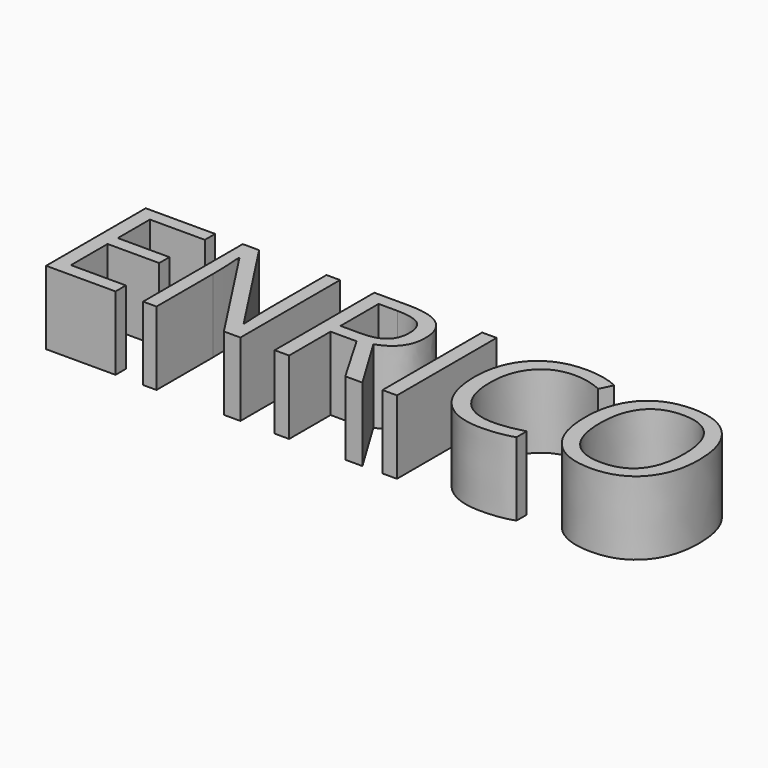
from build123d import *

# Parameters (mm, degrees)
F0_TEXT_SIZE = 60.3270251304
F1_DEPTH     = 25.4


# Not quite as in the source:
# - Text() gives the source's letters only with a copy of the font that has no kerning and outlines rounded to 1/6400 em; it was checked with that copy


with BuildPart() as f1:
    # F0 (on Top) → F1 (new body)
    with BuildSketch(Plane.XY):
        with Locations((-17.2073114663, -43.4354580939)):
            Text('ENRICO', F0_TEXT_SIZE, font='Open Sans', text_align=(TextAlign.LEFT, TextAlign.BOTTOM))
    extrude(amount=F1_DEPTH)


solid = f1.part
